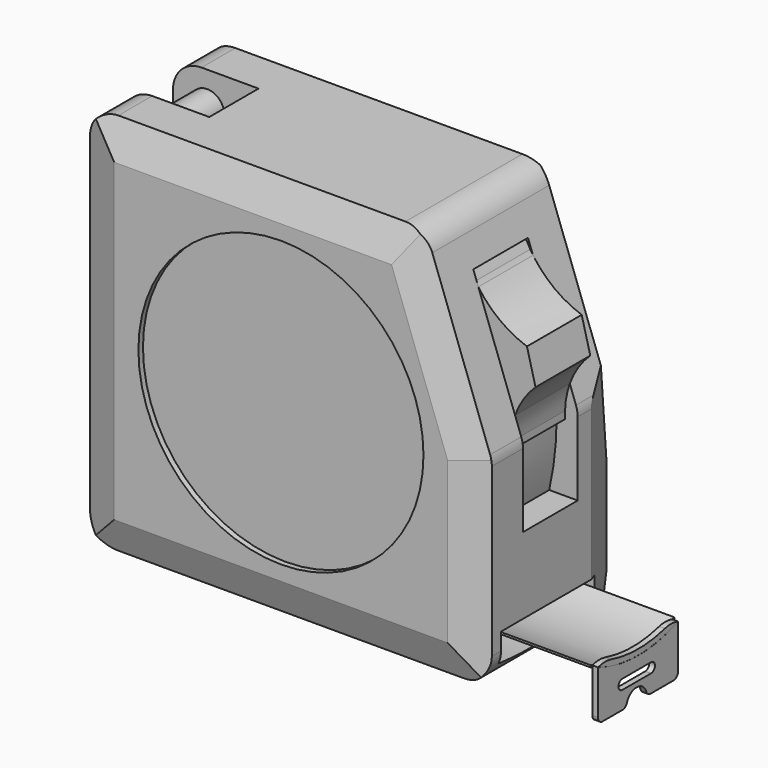
from build123d import *

# Parameters (mm, degrees)
F0_W          = 70.5
F0_H          = 67.2
F1_DEPTH      = 15
F2_SIZE2      = 11.6470474965
F2_SIZE       = 32
F3_R          = 25
F4_DEPTH      = 1
F6_DEPTH      = 6.6
F9_DEPTH      = 25
F10_C1_SIZE2  = 6
F10_C1_SIZE   = 2.1838214056
F10_C2_SIZE2  = 6
F10_C2_SIZE   = 2.1838214056
F10_C3_SIZE2  = 2.1838214056
F10_C3_SIZE   = 6
F10_C4_SIZE2  = 6
F10_C4_SIZE   = 2.1838214056
F10_C5_SIZE2  = 2.1838214056
F10_C5_SIZE   = 6
F10_C6_SIZE2  = 2.1838214056
F10_C6_SIZE   = 6
F10_C7_SIZE2  = 6
F10_C7_SIZE   = 2.1838214056
F10_C8_SIZE2  = 2.1838214056
F10_C8_SIZE   = 6
F10_C9_SIZE2  = 6
F10_C9_SIZE   = 2.1838214056
F10_C10_SIZE2 = 2.1838214056
F10_C10_SIZE  = 6
F11_R         = 5
F12_W         = 15
F12_H         = 15
F12_R         = 3
F13_DEPTH     = 5.4
F15_DEPTH     = 6
F16_DEPTH     = 6
F18_DEPTH     = 12.5
F20_DEPTH     = 50
F22_DEPTH     = 1
F23_T1_DEPTH  = 16.310631425
F23_T3_DEPTH  = 16.288826013
F24_R         = 1


# Not quite as in the source:
# - a fillet or chamfer that OpenCascade refuses, or shapes differently, is made with other operations: its cross-section is extruded or revolved along the edge and cut away or added


with BuildPart() as f1:
    # F0 (on Front) → F1 (new body, symmetric)
    with BuildSketch(Plane.XZ):
        Rectangle(F0_W, F0_H)
    extrude(amount=F1_DEPTH, both=True)

    # F2
    f2_edges = [f1.edges().sort_by_distance(p)[0] for p in [
        (35.25, 0, 33.6),
    ]]
    f2_side = f1.faces().sort_by_distance((35.25, 0, 0))[0]
    chamfer(f2_edges, length=F2_SIZE, length2=F2_SIZE2, reference=f2_side)

    # F3 (on face) → F4 (cut)
    with BuildSketch(Plane.XZ.offset(15)):
        Circle(F3_R)
    extrude(amount=-F4_DEPTH, mode=Mode.SUBTRACT)

    # F5 (on face) → F6 (join)
    with BuildSketch(Plane(origin=(0, 15, 0), x_dir=(-1, 0, 0), z_dir=(0, 1, 0))):
        with BuildLine():
            Line((12.25, 17.4), (-6.05, 17.4))
            Line((-6.05, 17.4), (-6.05, -12.6))
            ThreePointArc((-6.05, -12.6), (3.1, -18.6), (12.25, -12.6))
            Line((12.25, -12.6), (12.25, 17.4))
        make_face()
        with BuildLine():
            Line((5.9324988522, 8.8087505739), (5.9324988522, -3.8089272891))
            ThreePointArc((5.9324988522, -3.8089272891), (3.1412494261, -6.6001767152), (0.35, -3.8089272891))
            Line((0.35, -3.8089272891), (0.35, 8.8087505739))
            ThreePointArc((0.35, 8.8087505739), (3.1412494261, 11.6), (5.9324988522, 8.8087505739))
        make_face(mode=Mode.SUBTRACT)
    extrude(amount=F6_DEPTH)

    # F8 (on face) → F9 (cut)
    with BuildSketch(Plane.YZ.offset(6.05)):
        with BuildLine():
            Line((21.6, 14.4), (21.6, 17.4))
            Line((21.6, 17.4), (18.2999999846, 17.4))
            ThreePointArc((18.2999999846, 17.4), (20.5299103064, 16.5379013485), (21.6, 14.4))
        make_face()
        with BuildLine():
            Line((22.0904313028, -19.2825254053), (21.6, 14.4))
            Line((21.6, 14.4), (16.0833094269, -10.5487955734))
            ThreePointArc((16.0833094269, -10.5487955734), (15.9758103305, -12.88585804), (16.6612472385, -15.1227293536))
            Line((16.6612472385, -15.1227293536), (18.3251649141, -19.2825254053))
            Line((18.3251649141, -19.2825254053), (22.0904313028, -19.2825254053))
        make_face()
        with BuildLine():
            ThreePointArc((15, 14.4), (16.0700896822, 16.5379013381), (18.2999999846, 17.4))
            Line((18.2999999846, 17.4), (15, 17.4))
            Line((15, 17.4), (15, 14.4))
        make_face()
        with BuildLine():
            Line((15.5951015153, -10.4408427876), (21.0940559032, 14.427742295))
            ThreePointArc((21.0940559032, 14.427742295), (18.2621501284, 16.899744759), (15.497738322, 14.3524886147))
            Line((15.497738322, 14.3524886147), (15, -19.7163168341))
            Line((15, -19.7163168341), (17.8609258261, -19.4682209573))
            Line((17.8609258261, -19.4682209573), (16.2050844974, -15.328615782))
            ThreePointArc((16.2050844974, -15.328615782), (15.4783504264, -12.9373618021), (15.5951015153, -10.4408427876))
        make_face()
    extrude(amount=-F9_DEPTH, mode=Mode.SUBTRACT)

    # F10: chamfer of 6 x 2.1838214056 on 10 edges, made by hand

    # F10_c1
    f10_c1_edges = [f1.edges().sort_by_distance(p)[0] for p in [
        (-5.8235237483, 15, 33.6),
    ]]
    f10_c1_side = f1.faces().sort_by_distance((-5.8235237483, 14.9563235719, 33.6))[0]
    chamfer(f10_c1_edges, length=F10_C1_SIZE, length2=F10_C1_SIZE2, reference=f10_c1_side)

    # F10_c2
    f10_c2_edges = [f1.edges().sort_by_distance(p)[0] for p in [
        (-5.8235237483, -15, 33.6),
    ]]
    f10_c2_side = f1.faces().sort_by_distance((-5.8235237483, -14.9563235719, 33.6))[0]
    chamfer(f10_c2_edges, length=F10_C2_SIZE, length2=F10_C2_SIZE2, reference=f10_c2_side)

    # F10_c3
    f10_c3_edges = [f1.edges().sort_by_distance(p)[0] for p in [
        (35.25, -15, -16),
    ]]
    f10_c3_side = f1.faces().sort_by_distance((35.2063235719, -15, -16))[0]
    chamfer(f10_c3_edges, length=F10_C3_SIZE, length2=F10_C3_SIZE2, reference=f10_c3_side)

    # F10_c4
    f10_c4_edges = [f1.edges().sort_by_distance(p)[0] for p in [
        (27.5183869545, -15, 22.8424322584),
    ]]
    f10_c4_side = f1.faces().sort_by_distance((27.5183869545, -14.9563235719, 22.8424322584))[0]
    chamfer(f10_c4_edges, length=F10_C4_SIZE, length2=F10_C4_SIZE2, reference=f10_c4_side)

    # F10_c5
    f10_c5_edges = [f1.edges().sort_by_distance(p)[0] for p in [
        (-3, -15, -33.6),
    ]]
    f10_c5_side = f1.faces().sort_by_distance((-3, -15, -33.5563235719))[0]
    chamfer(f10_c5_edges, length=F10_C5_SIZE, length2=F10_C5_SIZE2, reference=f10_c5_side)

    # F10_c6
    f10_c6_edges = [f1.edges().sort_by_distance(p)[0] for p in [
        (-35.25, -15, 0),
    ]]
    f10_c6_side = f1.faces().sort_by_distance((-35.2063235719, -15, 0))[0]
    chamfer(f10_c6_edges, length=F10_C6_SIZE, length2=F10_C6_SIZE2, reference=f10_c6_side)

    # F10_c7
    f10_c7_edges = [f1.edges().sort_by_distance(p)[0] for p in [
        (0, 15, -33.6),
    ]]
    f10_c7_side = f1.faces().sort_by_distance((0, 14.9563235719, -33.6))[0]
    chamfer(f10_c7_edges, length=F10_C7_SIZE, length2=F10_C7_SIZE2, reference=f10_c7_side)

    # F10_c8
    f10_c8_edges = [f1.edges().sort_by_distance(p)[0] for p in [
        (35.25, 15, -13),
    ]]
    f10_c8_side = f1.faces().sort_by_distance((35.25, 14.9563235719, -13))[0]
    chamfer(f10_c8_edges, length=F10_C8_SIZE, length2=F10_C8_SIZE2, reference=f10_c8_side)

    # F10_c9
    f10_c9_edges = [f1.edges().sort_by_distance(p)[0] for p in [
        (-35.25, 15, 0),
    ]]
    f10_c9_side = f1.faces().sort_by_distance((-35.25, 14.9563235719, 0))[0]
    chamfer(f10_c9_edges, length=F10_C9_SIZE, length2=F10_C9_SIZE2, reference=f10_c9_side)

    # F10_c10
    f10_c10_edges = [f1.edges().sort_by_distance(p)[0] for p in [
        (29.4264762517, 15, 17.6),
    ]]
    f10_c10_side = f1.faces().sort_by_distance((29.3854338345, 15, 17.5850617818))[0]
    chamfer(f10_c10_edges, length=F10_C10_SIZE, length2=F10_C10_SIZE2, reference=f10_c10_side)

    # F11
    f11_edges = [f1.edges().sort_by_distance(p)[0] for p in [
        (-35.25, 0, 33.6),
        (23.602953, 0, 33.6),
        (35.25, -1.908089, 1.6),
        (35.25, -1.908089, -33.6),
        (-35.25, 0, -33.6),
    ]]
    fillet(f11_edges, radius=F11_R)

    # F12 (on Front) → F13 (cut, symmetric)
    with BuildSketch(Plane.XZ):
        with Locations((-27.75, 26.1)):
            Rectangle(F12_W, F12_H)
        with Locations((-29.25, 27.6)):
            Circle(F12_R, mode=Mode.SUBTRACT)
    extrude(amount=F13_DEPTH, both=True, mode=Mode.SUBTRACT)

    # F14 (on Front) → F15 (cut, symmetric)
    with BuildSketch(Plane.XZ):
        with BuildLine():
            Line((27.4193631632, 23.1144978891), (26.5368968656, 25.5390541151))
            Line((26.5368968656, 25.5390541151), (26.0889162393, 25.3760025016))
            ThreePointArc((26.0889162393, 25.3760025016), (26.5103242265, 24.6285041011), (26.9194386018, 23.8742070918))
            ThreePointArc((26.9194386018, 23.8742070918), (27.1643457119, 23.4910259493), (27.4193631632, 23.1144978891))
        make_face()
        with BuildLine():
            Line((35.25, 1.6), (33.866590897, 5.4008852724))
            ThreePointArc((33.866590897, 5.4008852724), (33.2694059355, 3.2061865059), (33.0300734223, 0.9443172563))
            ThreePointArc((33.0300734223, 0.9443172563), (33.0467289701, 0.3032247951), (33.0555394962, -0.3380234608))
            Line((33.0555394962, -0.3380234608), (31.5555830572, -0.3494550379))
            ThreePointArc((31.5555830572, -0.3494550379), (31.2508544156, -6.3130738574), (30.25, -12.2))
            Line((30.25, -12.2), (35.25, -12.2))
            Line((35.25, -12.2), (35.25, 1.6))
        make_face()
    extrude(amount=F15_DEPTH, both=True, mode=Mode.SUBTRACT)

    # F14 (on Front) → F16 (join, symmetric)
    with BuildSketch(Plane.XZ):
        with BuildLine():
            ThreePointArc((35.9503940222, 16.7019859811), (31.171399147, 19.2251228923), (27.4193631632, 23.1144978891))
            Line((27.4193631632, 23.1144978891), (27.695363868, 22.3561921849))
            Line((27.695363868, 22.3561921849), (33.866590897, 5.4008852724))
            ThreePointArc((33.866590897, 5.4008852724), (35.3399690851, 8.3575306064), (37.4562753297, 10.8940326852))
            Line((37.4562753297, 10.8940326852), (35.9503940222, 16.7019859811))
        make_face()
    extrude(amount=F16_DEPTH, both=True)

    # F17 (on face) → F18 (cut, symmetric)
    with BuildSketch(Plane.YZ.offset(35.25)):
        with BuildLine():
            Line((-10.8161785944, -25.6), (-10.8161785944, -30.691060879))
            ThreePointArc((-10.8161785944, -30.691060879), (-0.3161785944, -31.6), (10.1838214056, -30.691060879))
            Line((10.1838214056, -30.691060879), (10.1838214056, -25.6))
            Line((10.1838214056, -25.6), (-10.8161785944, -25.6))
        make_face()
    extrude(amount=F18_DEPTH, both=True, mode=Mode.SUBTRACT)

    # F19 (on Right) → F20 (join)
    with BuildSketch(Plane.YZ):
        with BuildLine():
            ThreePointArc((8.714591153, -26.5200827271), (-0.4161624238, -28.3920747054), (-9.5469160005, -26.5200827271))
            Line((-9.5469160005, -26.5200827271), (-9.6649662649, -26.7958799988))
            ThreePointArc((-9.6649662649, -26.7958799988), (-0.4161624238, -28.6920747054), (8.8326414173, -26.7958799988))
            Line((8.8326414173, -26.7958799988), (8.714591153, -26.5200827271))
        make_face()
    extrude(amount=F20_DEPTH)

    # F21 (on face) → F22 (join)
    with BuildSketch(Plane.YZ.offset(50)):
        with BuildLine():
            ThreePointArc((8.3190464543, -27.0085648953), (-0.4562043728, -28.692040597), (-9.2256682302, -26.9786751448))
            Line((-9.2256682302, -26.9786751448), (-9.2256682302, -35.402658417))
            Line((-9.2256682302, -35.402658417), (-3.023406025, -35.402658417))
            ThreePointArc((-3.023406025, -35.402658417), (-0.7754032849, -33.1676302601), (1.4725994552, -35.402658417))
            Line((1.4725994552, -35.402658417), (8.3190464543, -35.402658417))
            Line((8.3190464543, -35.402658417), (8.3190464543, -27.0085648953))
        make_face()
        with BuildLine():
            ThreePointArc((-3.8824020182, -32.2988011143), (-4.7451472338, -31.4360558987), (-3.8824020182, -30.573310683))
            Line((-3.8824020182, -30.573310683), (2.3921075505, -30.573310683))
            ThreePointArc((2.3921075505, -30.573310683), (3.2548527662, -31.4360558987), (2.3921075505, -32.2988011143))
            Line((2.3921075505, -32.2988011143), (-3.8824020182, -32.2988011143))
        make_face(mode=Mode.SUBTRACT)
        with BuildLine():
            ThreePointArc((8.3190464543, -26.686091106), (-0.4563238607, -28.4026234806), (-9.2256682302, -26.6555668451))
            Line((-9.2256682302, -26.6555668451), (-9.2256682302, -26.9786751448))
            ThreePointArc((-9.2256682302, -26.9786751448), (-0.4562043728, -28.692040597), (8.3190464543, -27.0085648953))
            Line((8.3190464543, -27.0085648953), (8.3190464543, -26.686091106))
        make_face()
    extrude(amount=F22_DEPTH)

    # F24
    f24_edges = [f1.edges().sort_by_distance(p)[0] for p in [
        (50.5, -9.225668, -35.402658),
        (50.5, 8.319046, -35.402658),
        (50.5, 1.472599, -35.402658),
        (50.5, -3.023406, -35.402658),
    ]]
    fillet(f24_edges, radius=F24_R)


with BuildPart() as f22:
    # F21 (on face) → F22, piece 2 (new body)
    with BuildSketch(Plane.YZ.offset(50)):
        with BuildLine():
            Line((-9.2256682302, -25.5694771946), (-9.2256682302, -26.6547433463))
            ThreePointArc((-9.2256682302, -26.6547433463), (-0.4562889695, -28.3920400099), (8.3190464543, -26.6850835031))
            Line((8.3190464543, -26.6850835031), (8.3190464543, -25.6016359995))
            ThreePointArc((8.3190464543, -25.6016359995), (-0.4566414995, -27.4026213187), (-9.2256682302, -25.5694771946))
        make_face()
    extrude(amount=F22_DEPTH)

    # F23: fillet of radius 5 on 2 edges, made by hand

    # F23_s2 → F23_t1 (cut)
    with BuildSketch(Plane.YZ.offset(42.3446842875)):
        with BuildLine():
            ThreePointArc((-6.3397976534, -26.5933758219), (-7.7872577117, -26.4112776514), (-9.2256682302, -26.6547433463))
            Line((-9.2256682302, -26.6547433463), (-9.2256682302, -25.5694771946))
            ThreePointArc((-9.2256682302, -25.5694771946), (-7.8005008028, -26.131505438), (-6.3397976534, -26.5933758219))
        make_face()
    extrude(amount=F23_T1_DEPTH, mode=Mode.SUBTRACT)

    # F23_s4 → F23_t3 (cut)
    with BuildSketch(Plane.YZ.offset(42.3555869935)):
        with BuildLine():
            ThreePointArc((8.3190464543, -26.6850835031), (6.8816079641, -26.4367102191), (5.4336572883, -26.6137908268))
            ThreePointArc((5.4336572883, -26.6137908268), (6.8938908655, -26.1577125068), (8.3190464543, -25.6016359995))
            Line((8.3190464543, -25.6016359995), (8.3190464543, -26.6850835031))
        make_face()
    extrude(amount=F23_T3_DEPTH, mode=Mode.SUBTRACT)


solid = Compound([f1.part, f22.part])
